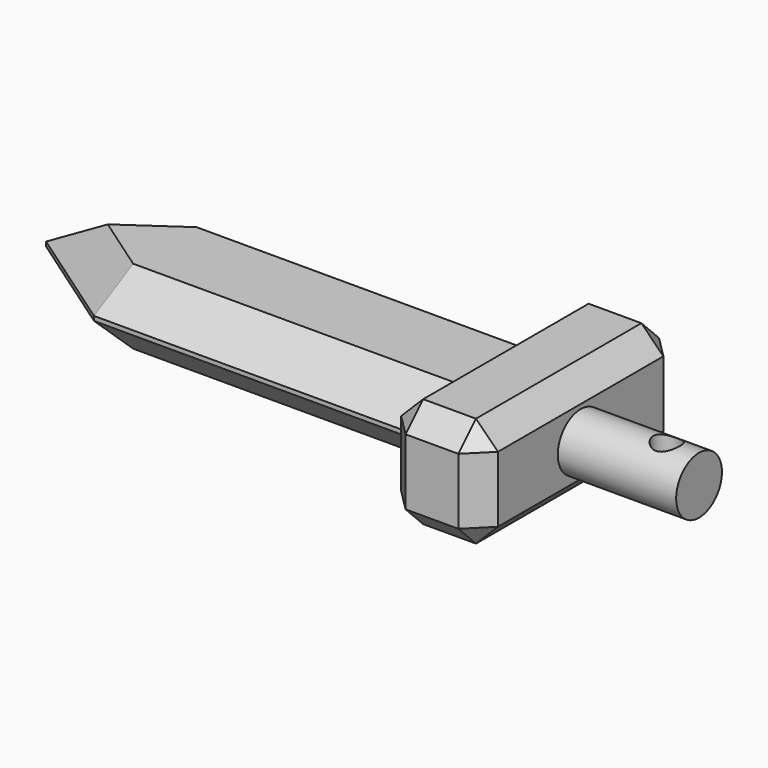
from build123d import *

# Parameters (mm, degrees)
F1_DEPTH     = 12.5
F2_DEPTH     = 8.5
F3_SIZE      = 8
F4_T1_DEPTH  = 6.3508529611
F4_T3_DEPTH  = 6.3508529611
F4_T5_DEPTH  = 6.3508529611
F4_T7_DEPTH  = 6.3508529611
F4_T9_DEPTH  = 6.3508529611
F4_T11_DEPTH = 6.3508529611
F4_T13_DEPTH = 6.3508529611
F4_T15_DEPTH = 6.3508529611
F4_T17_DEPTH = 50.7168298797
F4_T19_DEPTH = 47.7168298797
F4_T21_DEPTH = 82.7168298797
F4_T26_DEPTH = 82.7168298797
F4_T31_DEPTH = 82.7168298797
F4_T36_DEPTH = 82.7168298797
F4_T41_DEPTH = 82.7168298797
F4_T46_DEPTH = 82.7168298797
F4_T51_DEPTH = 82.7168298797
F5_R         = 6.5
F6_DEPTH     = 26.9
F7_R         = 3.0614301368
F8_DEPTH     = 6.5


# Not quite as in the source:
# - a fillet or chamfer that OpenCascade refuses, or shapes differently, is made with other operations: its cross-section is extruded or revolved along the edge and cut away or added


with BuildPart() as f1:
    # F0 (on Top) → F1 (new body, symmetric)
    with BuildSketch(Plane.XY):
        Polygon((25.0318072736, -28.5), (47.0318072736, -28.5), (47.0318072736, 0), (47.0318072736, 28.5), (25.0318072736, 28.5), (25.0318072736, 17), (25.0318072736, -17), align=None)
    extrude(amount=F1_DEPTH, both=True)

    # F0 (on Top) → F2 (join, symmetric)
    with BuildSketch(Plane.XY):
        Polygon((-49.9681927264, -17), (25.0318072736, -17), (25.0318072736, 17), (-49.9681927264, 17), (-74.4579061866, 0), align=None)
    extrude(amount=F2_DEPTH, both=True)

    # F3
    f3_edges = [f1.edges().sort_by_distance(p)[0] for p in [
        (-12.468193, 17, -8.5),
        (-12.468193, -17, -8.5),
        (-62.213049, -8.5, -8.5),
        (-12.468193, -17, 8.5),
        (-12.468193, 17, 8.5),
        (-62.213049, -8.5, 8.5),
        (-62.213049, 8.5, 8.5),
        (-62.213049, 8.5, -8.5),
    ]]
    chamfer(f3_edges, length=F3_SIZE)

    # F4: chamfer of 5 on 12 edges, made by hand

    # F4_s2 → F4_t1 (cut)
    with BuildSketch(Plane(origin=(-1.9893975755, 1.9893975755, -1.9893975755), x_dir=(-0.7071067812, -0.7071067812, 0), z_dir=(-0.5773502692, 0.5773502692, -0.5773502692))):
        Polygon((-34.3171700264, -6.7490820577), (-37.8527039324, -12.8728064147), (-41.3882378383, -6.7490820577), align=None)
    extrude(amount=F4_T1_DEPTH, mode=Mode.SUBTRACT)

    # F4_s4 → F4_t3 (cut)
    with BuildSketch(Plane(origin=(-1.9893975755, -1.9893975755, -1.9893975755), x_dir=(0.7071067812, -0.7071067812, 0), z_dir=(-0.5773502692, -0.5773502692, -0.5773502692))):
        Polygon((34.3171700264, -6.7490820577), (41.3882378383, -6.7490820577), (37.8527039324, -12.8728064147), align=None)
    extrude(amount=F4_T3_DEPTH, mode=Mode.SUBTRACT)

    # F4_s6 → F4_t5 (cut)
    with BuildSketch(Plane(origin=(-1.9893975755, -1.9893975755, 1.9893975755), x_dir=(0.7071067812, -0.7071067812, 0), z_dir=(-0.5773502692, -0.5773502692, 0.5773502692))):
        Polygon((34.3171700264, 6.7490820577), (41.3882378383, 6.7490820577), (37.8527039324, 12.8728064147), align=None)
    extrude(amount=F4_T5_DEPTH, mode=Mode.SUBTRACT)

    # F4_s8 → F4_t7 (cut)
    with BuildSketch(Plane(origin=(-1.9893975755, 1.9893975755, 1.9893975755), x_dir=(-0.7071067812, -0.7071067812, 0), z_dir=(-0.5773502692, 0.5773502692, 0.5773502692))):
        Polygon((-34.3171700264, 6.7490820577), (-37.8527039324, 12.8728064147), (-41.3882378383, 6.7490820577), align=None)
    extrude(amount=F4_T7_DEPTH, mode=Mode.SUBTRACT)

    # F4_s10 → F4_t9 (cut)
    with BuildSketch(Plane(origin=(26.0106024245, 26.0106024245, -26.0106024245), x_dir=(-0.7071067812, 0.7071067812, 0), z_dir=(0.5773502692, 0.5773502692, -0.5773502692))):
        Polygon((-16.6395004968, 22.6707653858), (-13.1039665908, 16.5470410289), (-9.5684326849, 22.6707653858), align=None)
    extrude(amount=F4_T9_DEPTH, mode=Mode.SUBTRACT)

    # F4_s12 → F4_t11 (cut)
    with BuildSketch(Plane(origin=(26.0106024245, 26.0106024245, 26.0106024245), x_dir=(-0.7071067812, 0.7071067812, 0), z_dir=(0.5773502692, 0.5773502692, 0.5773502692))):
        Polygon((-13.1039665908, -16.5470410289), (-16.6395004968, -22.6707653858), (-9.5684326849, -22.6707653858), align=None)
    extrude(amount=F4_T11_DEPTH, mode=Mode.SUBTRACT)

    # F4_s14 → F4_t13 (cut)
    with BuildSketch(Plane(origin=(26.0106024245, -26.0106024245, -26.0106024245), x_dir=(0.7071067812, 0.7071067812, 0), z_dir=(0.5773502692, -0.5773502692, -0.5773502692))):
        Polygon((16.6395004968, 22.6707653858), (9.5684326849, 22.6707653858), (13.1039665908, 16.5470410289), align=None)
    extrude(amount=F4_T13_DEPTH, mode=Mode.SUBTRACT)

    # F4_s16 → F4_t15 (cut)
    with BuildSketch(Plane(origin=(26.0106024245, -26.0106024245, 26.0106024245), x_dir=(0.7071067812, 0.7071067812, 0), z_dir=(0.5773502692, -0.5773502692, 0.5773502692))):
        Polygon((9.5684326849, -22.6707653858), (13.1039665908, -16.5470410289), (16.6395004968, -22.6707653858), align=None)
    extrude(amount=F4_T15_DEPTH, mode=Mode.SUBTRACT)

    # F4_s18 → F4_t17 (cut)
    with BuildSketch(Plane.XY.offset(-25.3584149398)):
        Polygon((25.0318072736, -23.5), (30.0318072736, -28.5), (25.0318072736, -28.5), align=None)
        Polygon((25.0318072736, 23.5), (30.0318072736, 28.5), (25.0318072736, 28.5), align=None)
        Polygon((42.0318072736, 28.5), (47.0318072736, 23.5), (47.0318072736, 28.5), align=None)
        Polygon((42.0318072736, -28.5), (47.0318072736, -23.5), (47.0318072736, -28.5), align=None)
    extrude(amount=F4_T17_DEPTH, mode=Mode.SUBTRACT)

    # F4_s20 → F4_t19 (cut)
    with BuildSketch(Plane.YZ.offset(12.1733923338)):
        Polygon((23.5, -12.5), (28.5, -7.5), (28.5, -12.5), align=None)
        Polygon((23.5, 12.5), (28.5, 7.5), (28.5, 12.5), align=None)
        Polygon((-28.5, -7.5), (-23.5, -12.5), (-28.5, -12.5), align=None)
        Polygon((-28.5, 7.5), (-23.5, 12.5), (-28.5, 12.5), align=None)
    extrude(amount=F4_T19_DEPTH, mode=Mode.SUBTRACT)

    # F4_s22 → F4_t21 (cut)
    with BuildSketch(Plane.XZ.offset(-41.3584149398)):
        Polygon((42.0318072736, 12.5), (47.0318072736, 7.5), (47.0318072736, 12.5), align=None)
        Polygon((42.0318072736, -12.5), (47.0318072736, -7.5), (47.0318072736, -12.5), align=None)
    extrude(amount=F4_T21_DEPTH, mode=Mode.SUBTRACT)


with BuildPart() as f4_tool24:
    # F4_s25 → F4_t26 (new body)
    with BuildSketch(Plane.XZ.offset(-41.3584149398)):
        Polygon((25.0318072736, -7.5), (30.0318072736, -12.5), (25.0318072736, -12.5), align=None)
    extrude(amount=F4_T26_DEPTH)

    split(bisect_by=Plane(origin=(0, 8.75, -8.75), x_dir=(1, 0, 0), z_dir=(0, 0.7071067812, -0.7071067812)), keep=Keep.TOP)


with BuildPart() as f1_1:
    add(f1.part)

    # F4_t23: cut F4_tool24
    add(f4_tool24.part, mode=Mode.SUBTRACT)


with BuildPart() as f4_tool29:
    # F4_s30 → F4_t31 (new body)
    with BuildSketch(Plane.XZ.offset(-41.3584149398)):
        Polygon((25.0318072736, -7.5), (30.0318072736, -12.5), (25.0318072736, -12.5), align=None)
    extrude(amount=F4_T31_DEPTH)

    split(bisect_by=Plane.XY.offset(-8.5), keep=Keep.BOTTOM)


with BuildPart() as f1_2:
    add(f1_1.part)

    # F4_t28: cut F4_tool29
    add(f4_tool29.part, mode=Mode.SUBTRACT)


with BuildPart() as f4_tool34:
    # F4_s35 → F4_t36 (new body)
    with BuildSketch(Plane.XZ.offset(-41.3584149398)):
        Polygon((25.0318072736, -7.5), (30.0318072736, -12.5), (25.0318072736, -12.5), align=None)
    extrude(amount=F4_T36_DEPTH)

    split(bisect_by=Plane(origin=(0, -8.75, -8.75), x_dir=(1, 0, 0), z_dir=(0, -0.7071067812, -0.7071067812)), keep=Keep.TOP)


with BuildPart() as f1_3:
    add(f1_2.part)

    # F4_t33: cut F4_tool34
    add(f4_tool34.part, mode=Mode.SUBTRACT)


with BuildPart() as f4_tool39:
    # F4_s40 → F4_t41 (new body)
    with BuildSketch(Plane.XZ.offset(41.3584149398)):
        Polygon((25.0318072736, 7.5), (30.0318072736, 12.5), (25.0318072736, 12.5), align=None)
    extrude(amount=-F4_T41_DEPTH)

    split(bisect_by=Plane(origin=(0, -8.75, 8.75), x_dir=(1, 0, 0), z_dir=(0, -0.7071067812, 0.7071067812)), keep=Keep.TOP)


with BuildPart() as f1_4:
    add(f1_3.part)

    # F4_t38: cut F4_tool39
    add(f4_tool39.part, mode=Mode.SUBTRACT)


with BuildPart() as f4_tool44:
    # F4_s45 → F4_t46 (new body)
    with BuildSketch(Plane.XZ.offset(41.3584149398)):
        Polygon((25.0318072736, 7.5), (30.0318072736, 12.5), (25.0318072736, 12.5), align=None)
    extrude(amount=-F4_T46_DEPTH)

    split(bisect_by=Plane.XY.offset(8.5), keep=Keep.TOP)


with BuildPart() as f1_5:
    add(f1_4.part)

    # F4_t43: cut F4_tool44
    add(f4_tool44.part, mode=Mode.SUBTRACT)


with BuildPart() as f4_tool49:
    # F4_s50 → F4_t51 (new body)
    with BuildSketch(Plane.XZ.offset(41.3584149398)):
        Polygon((25.0318072736, 7.5), (30.0318072736, 12.5), (25.0318072736, 12.5), align=None)
    extrude(amount=-F4_T51_DEPTH)

    split(bisect_by=Plane(origin=(0, 8.75, 8.75), x_dir=(1, 0, 0), z_dir=(0, 0.7071067812, 0.7071067812)), keep=Keep.TOP)


with BuildPart() as f1_6:
    add(f1_5.part)

    # F4_t48: cut F4_tool49
    add(f4_tool49.part, mode=Mode.SUBTRACT)

    # F5 (on face) → F6 (join)
    with BuildSketch(Plane.YZ.offset(47.0318072736)):
        Circle(F5_R)
    extrude(amount=F6_DEPTH)

    # F7 (on Top) → F8 (cut, symmetric)
    with BuildSketch(Plane.XY):
        with Locations((66.6042044759, 0)):
            Circle(F7_R)
    extrude(amount=F8_DEPTH, both=True, mode=Mode.SUBTRACT)


solid = f1_6.part
